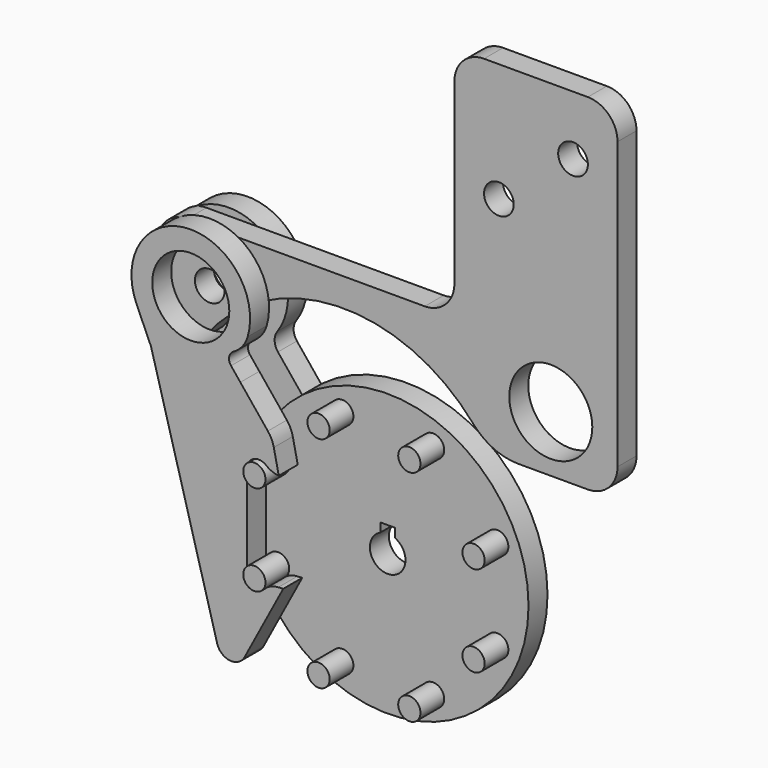
from build123d import *

# Parameters (mm, degrees)
F0_R          = 47.5
F1_DEPTH      = 5
F1_DEPTH_BACK = 3
F2_R          = 3.75
F3_DEPTH      = 10
F5_R          = 5
F5_R_2        = 14
F6_DEPTH      = 8
F7_R          = 13
F8_DEPTH      = 8
F11_R         = 13
F12_DEPTH     = 8
F13_R         = 13
F14_DEPTH     = 8
F16_DEPTH     = 25


with BuildPart() as f1:
    # F0 (on Front) → F1 (new body, two sides)
    with BuildSketch(Plane.XZ) as f1_sk:
        Circle(F0_R)
        with BuildLine():
            ThreePointArc((2.5, 5.4543560573), (0, -6), (-2.5, 5.4543560573))
            Line((-2.5, 5.4543560573), (-2.5, 8.5))
            Line((-2.5, 8.5), (2.5, 8.5))
            Line((2.5, 8.5), (2.5, 5.4543560573))
        make_face(mode=Mode.SUBTRACT)
    extrude(amount=F1_DEPTH)
    extrude(f1_sk.sketch, amount=-F1_DEPTH_BACK)

    # F2 (on face) → F3 (join)
    with BuildSketch(Plane.XZ.offset(5)):
        with Locations((15.3073372946, 36.9551813005)):
            Circle(F2_R)
        with Locations((-15.3073372946, 36.9551813005)):
            Circle(F2_R)
        with Locations((-36.9551813005, 15.3073372946)):
            Circle(F2_R)
        with Locations((-36.9551813005, -15.3073372946)):
            Circle(F2_R)
        with Locations((-15.3073372946, -36.9551813005)):
            Circle(F2_R)
        with Locations((15.3073372946, -36.9551813005)):
            Circle(F2_R)
        with Locations((36.9551813005, -15.3073372946)):
            Circle(F2_R)
        with Locations((36.9551813005, 15.3073372946)):
            Circle(F2_R)
    extrude(amount=F3_DEPTH)


with BuildPart() as f6:
    # F5 (on face) → F6 (new body)
    with BuildSketch(Plane.XZ.offset(5)):
        with BuildLine():
            ThreePointArc((32.5, 157.5), (25.4289321881, 154.5710678119), (22.5, 147.5))
            Line((22.5, 147.5), (22.5, 87.5))
            ThreePointArc((22.5, 87.5), (19.5710678119, 80.4289321881), (12.5, 77.5))
            Line((12.5, 77.5), (-67.5, 77.5))
            ThreePointArc((-67.5, 77.5), (-74.5710678119, 74.5710678119), (-77.5, 67.5))
            Line((-77.5, 67.5), (-77.5, 52.5))
            ThreePointArc((-77.5, 52.5), (-74.5710678119, 45.4289321881), (-67.5, 42.5))
            Line((-67.5, 42.5), (-65.6236110921, 42.5))
            ThreePointArc((-65.6236110921, 42.5), (-63.374272565, 43.0345239682), (-61.60586418, 44.5238095238))
            ThreePointArc((-61.60586418, 44.5238095238), (-17.1772348514, 67.9591204937), (28.884396278, 47.9230769231))
            ThreePointArc((28.884396278, 47.9230769231), (35.6964437753, 42.8129378192), (44.0169467187, 41))
            Line((44.0169467187, 41), (67.5, 41))
            ThreePointArc((67.5, 41), (74.5710678119, 43.9289321881), (77.5, 51))
            Line((77.5, 51), (77.5, 147.5))
            ThreePointArc((77.5, 147.5), (74.5710678119, 154.5710678119), (67.5, 157.5))
            Line((67.5, 157.5), (32.5, 157.5))
        make_face()
        with Locations((-60, 60)):
            Circle(F5_R, mode=Mode.SUBTRACT)
        with Locations((55, 60)):
            Circle(F5_R_2, mode=Mode.SUBTRACT)
        with Locations((37.5, 117.5)):
            Circle(F5_R, mode=Mode.SUBTRACT)
        with Locations((62.5, 137.5)):
            Circle(F5_R, mode=Mode.SUBTRACT)
    extrude(amount=-F6_DEPTH)


with BuildPart() as f8:
    # F7 (on face) → F8 (new body)
    with BuildSketch(Plane.XZ.offset(5)):
        with BuildLine():
            Line((-45.5454252447, 5.6539239871), (-42.0390263481, 58.8153374007))
            ThreePointArc((-42.0390263481, 58.8153374007), (-61.8254025331, 77.9072026177), (-77.3525061409, 55.21559506))
            Line((-77.3525061409, 55.21559506), (-51.0893218746, -40.0380617645))
            ThreePointArc((-51.0893218746, -40.0380617645), (-46.817223508, -43.6789346076), (-41.8544433156, -41.0564182062))
            Line((-41.8544433156, -41.0564182062), (-28.8216980003, -16.5453891757))
            Line((-28.8216980003, -16.5453891757), (-30.4861678116, -16.6331144374))
            ThreePointArc((-30.4861678116, -16.6331144374), (-32.6771791019, -17.0825556032), (-34.638229912, -18.1581054885))
            ThreePointArc((-34.638229912, -18.1581054885), (-38.5124264489, -18.7052097863), (-41, -15.6851601597))
            Line((-41, -15.6851601597), (-41, -1.6851601597))
            Line((-41, -1.6851601597), (-45.5454252447, 5.6539239871))
        make_face()
        with Locations((-60, 60)):
            Circle(F7_R, mode=Mode.SUBTRACT)
    extrude(amount=F8_DEPTH)

    # F13 (on face) → F14 (join)
    with BuildSketch(Plane(origin=(0, -5, 0), x_dir=(-1, 0, 0), z_dir=(0, 1, 0))):
        with BuildLine():
            Line((48.8274879805, -14.4962734092), (78.2813984598, 51.8888675048))
            ThreePointArc((78.2813984598, 51.8888675048), (57.4771635507, 79.8402443596), (44.3303405904, 47.5717348762))
            ThreePointArc((44.3303405904, 47.5717348762), (45.4128615623, 44.4393357528), (44.2986555453, 41.31806664))
            Line((44.2986555453, 41.31806664), (34.003863851, 28.6050576495))
            ThreePointArc((34.003863851, 28.6050576495), (32.7489738734, 26.6159230972), (31.9933678596, 24.3887130319))
            Line((31.9933678596, 24.3887130319), (30.3260801171, 16.5358292403))
            Line((30.3260801171, 16.5358292403), (30.4577421115, 16.5477985125))
            ThreePointArc((30.4577421115, 16.5477985125), (32.6300949094, 17.0801622574), (34.5488643782, 18.2294453214))
            ThreePointArc((34.5488643782, 18.2294453214), (38.3994763606, 18.9233540189), (41, 16))
            Line((41, 16), (41, -15.6851601597))
            Line((41, -15.6851601597), (46.9993481346, -15.6851601597))
            ThreePointArc((46.9993481346, -15.6851601597), (48.0897089695, -15.3617976427), (48.8274879805, -14.4962734092))
        make_face()
        with Locations((60, 60)):
            Circle(F13_R, mode=Mode.SUBTRACT)
    extrude(amount=-F14_DEPTH)

    # F15 (on face) → F16 (cut)
    with BuildSketch(Plane.XZ.offset(13)):
        with BuildLine():
            Line((-46.4229721787, 43.9413792102), (-43.2763702235, 40.0556494029))
            Line((-43.2763702235, 40.0556494029), (-35.2763702235, 40.0556494029))
            Line((-35.2763702235, 40.0556494029), (-35.2763702235, 54.3906954695))
            Line((-35.2763702235, 54.3906954695), (-40.8027162681, 54.3906954695))
            ThreePointArc((-40.8027162681, 54.3906954695), (-42.5889409712, 50.953061449), (-45.5476474881, 48.4522651567))
            ThreePointArc((-45.5476474881, 48.4522651567), (-47.0365994546, 46.4008219683), (-46.4229721787, 43.9413792102))
        make_face()
    extrude(amount=-F16_DEPTH, mode=Mode.SUBTRACT)


with BuildPart() as f12:
    # F11 (on face) → F12 (new body)
    with BuildSketch(Plane(origin=(0, 3, 0), x_dir=(-1, 0, 0), z_dir=(0, 1, 0))):
        with BuildLine():
            Line((49.0952220718, 8.375765293), (76.5411496684, 48.7576529298))
            ThreePointArc((76.5411496684, 48.7576529298), (59.8622252185, 79.9995254471), (43.615307759, 48.530830014))
            ThreePointArc((43.615307759, 48.530830014), (44.5160762599, 45.4886803355), (43.404864506, 42.5169355623))
            Line((43.404864506, 42.5169355623), (33.7035274984, 30.536782077))
            ThreePointArc((33.7035274984, 30.536782077), (32.4874272694, 28.6280699339), (31.7316772086, 26.4947805356))
            Line((31.7316772086, 26.4947805356), (30, 19))
            Line((30, 19), (43, 20))
            Line((43, 20), (41, 7.5))
            Line((41, 7.5), (47.441107105, 7.5))
            ThreePointArc((47.441107105, 7.5), (48.3769304286, 7.7324495178), (49.0952220718, 8.375765293))
        make_face()
        with Locations((60, 60)):
            Circle(F11_R, mode=Mode.SUBTRACT)
    extrude(amount=F12_DEPTH)


solid = Compound([f1.part, f6.part, f8.part, f12.part])
